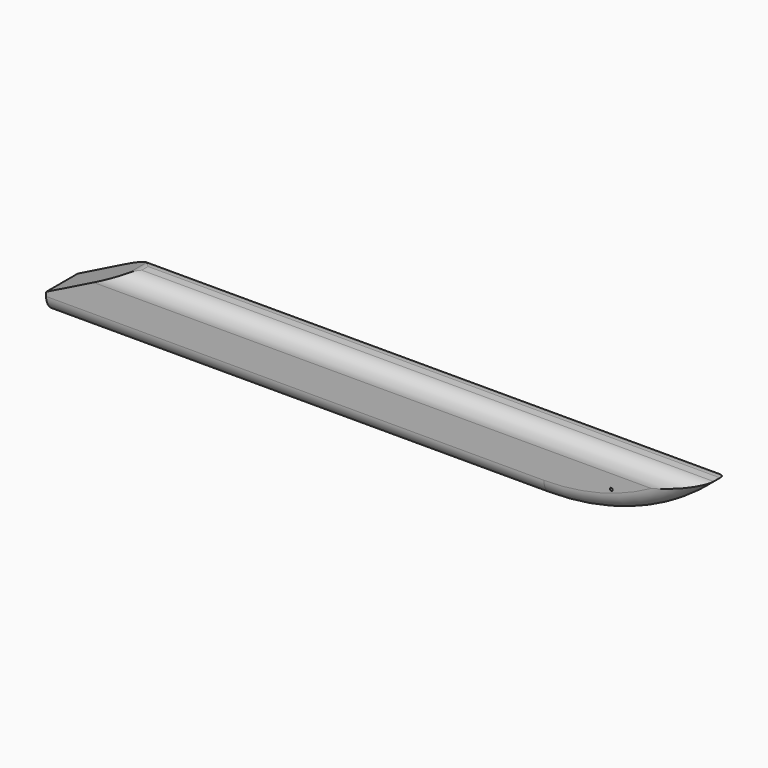
from build123d import *

# Parameters (mm, degrees)
F0_W        = 209.9508528371
F0_H        = 19.0544301776
F0_R        = 0.4554012186
F1_DEPTH    = 12.7
F2_T1_DEPTH = 264.7329269001
F3_SIZE2    = 25.4
F3_SIZE     = 12.7
F4_R        = 5.08


# Not quite as in the source:
# - a fillet or chamfer that OpenCascade refuses, or shapes differently, is made with other operations: its cross-section is extruded or revolved along the edge and cut away or added


with BuildPart() as f1:
    # F0 (on Front) → F1 (new body)
    with BuildSketch(Plane.XZ):
        Rectangle(F0_W, F0_H)
        with Locations((76.2023702264, 0)):
            Circle(F0_R, mode=Mode.SUBTRACT)
    extrude(amount=F1_DEPTH)

    # F2: fillet of radius 76.2 on 1 edges, made by hand

    # F2_s2 → F2_t1 (cut)
    with BuildSketch(Plane.XZ.offset(-126.0164634501)):
        with BuildLine():
            ThreePointArc((54.5688410385, -9.5272150888), (81.5127418283, -4.6046042822), (104.9754264186, 9.5272150888))
            Line((104.9754264186, 9.5272150888), (104.9754264186, -9.5272150888))
            Line((104.9754264186, -9.5272150888), (54.5688410385, -9.5272150888))
        make_face()
    extrude(amount=F2_T1_DEPTH, mode=Mode.SUBTRACT)

    # F3
    f3_edges = [f1.edges().sort_by_distance(p)[0] for p in [
        (-104.975426, -6.35, 9.527215),
    ]]
    f3_side = f1.faces().sort_by_distance((-104.975426, -6.35, 0))[0]
    chamfer(f3_edges, length=F3_SIZE, length2=F3_SIZE2, reference=f3_side)

    # F4
    f4_edges = [f1.edges().sort_by_distance(p)[0] for p in [
        (81.512742, -12.7, -4.604604),
        (12.7, -12.7, 9.527215),
        (12.7, 0, 9.527215),
        (-25.203293, 0, -9.527215),
        (-79.575426, -6.35, 9.527215),
        (-25.203293, -12.7, -9.527215),
        (81.512742, 0, -4.604604),
    ]]
    fillet(f4_edges, radius=F4_R)


solid = f1.part
